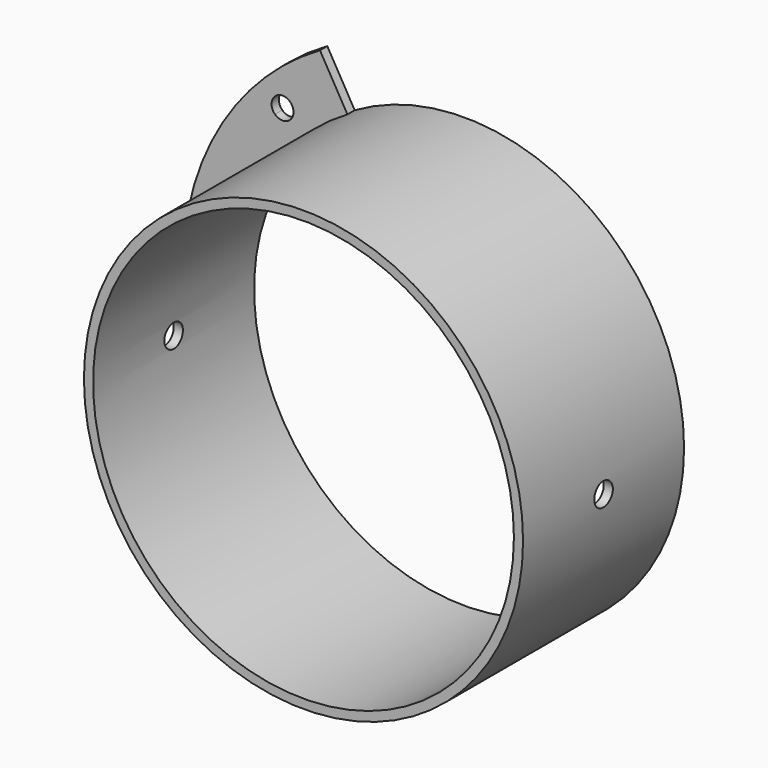
from build123d import *

# Parameters (mm, degrees)
F0_R     = 120
F0_R_2   = 115
F1_DEPTH = 55
F3_DEPTH = 5
F5_DEPTH = 110.001
F6_R     = 6.35
F7_DEPTH = 254


# Not quite as in the source:
# - a pattern or mirror of a feature is missing from the dataset's text; its kind, count and spacing are read off the source's solid


with BuildPart() as f1:
    # F0 (on Front) → F1 (new body, symmetric)
    with BuildSketch(Plane.XZ):
        Circle(F0_R)
        Circle(F0_R_2, mode=Mode.SUBTRACT)
    extrude(amount=F1_DEPTH, both=True)

    # F2 (on face) → F3 (join)
    with BuildSketch(Plane(origin=(0, 55, 0), x_dir=(-1, 0, 0), z_dir=(0, 1, 0))):
        with BuildLine():
            Line((60, -103.9230484541), (75, -129.9038105677))
            ThreePointArc((75, -129.9038105677), (150, 0), (75, 129.9038105677))
            Line((75, 129.9038105677), (60, 103.9230484541))
            ThreePointArc((60, 103.9230484541), (103.9230484541, 60), (120, 0))
            ThreePointArc((120, 0), (103.9230484541, -60), (60, -103.9230484541))
        make_face()
    extrude(amount=-F3_DEPTH)

    # F4 (on face) → F5 (cut, through all)
    with BuildSketch(Plane(origin=(0, 55, 0), x_dir=(-1, 0, 0), z_dir=(0, 1, 0))):
        with BuildLine():
            ThreePointArc((134.8666666667, 5.9985183356), (134.9666625504, 3), (135, 0))
            ThreePointArc((135, 0), (134.9666625504, -3), (134.8666666667, -5.9985183356))
            ThreePointArc((134.8666666667, -5.9985183356), (139.1952353927, -4.2895221179), (141, 0))
            ThreePointArc((141, 0), (139.1952353927, 4.2895221179), (134.8666666667, 5.9985183356))
        make_face()
        with BuildLine():
            ThreePointArc((134.8666666667, -5.9985183356), (134.9666625504, -3), (135, 0))
            ThreePointArc((135, 0), (134.9666625504, 3), (134.8666666667, 5.9985183356))
            ThreePointArc((134.8666666667, 5.9985183356), (129, 0), (134.8666666667, -5.9985183356))
        make_face()
    f5 = extrude(amount=-F5_DEPTH, mode=Mode.SUBTRACT)

    # F5_copies: F5 across plane
    add(f5.mirror(Plane(origin=(0, 0, 0), x_dir=(-0.9238795325, 0, -0.3826834324), z_dir=(0.3826834324, 0, -0.9238795325))), mode=Mode.SUBTRACT)

    # F5_copies1: F5 across plane
    add(f5.mirror(Plane(origin=(0, 0, 0), x_dir=(0.9238795325, 0, -0.3826834324), z_dir=(0.3826834324, 0, 0.9238795325))), mode=Mode.SUBTRACT)

    # F6 (on Right) → F7 (cut, symmetric)
    with BuildSketch(Plane.YZ):
        Circle(F6_R)
    extrude(amount=F7_DEPTH, both=True, mode=Mode.SUBTRACT)


solid = f1.part
